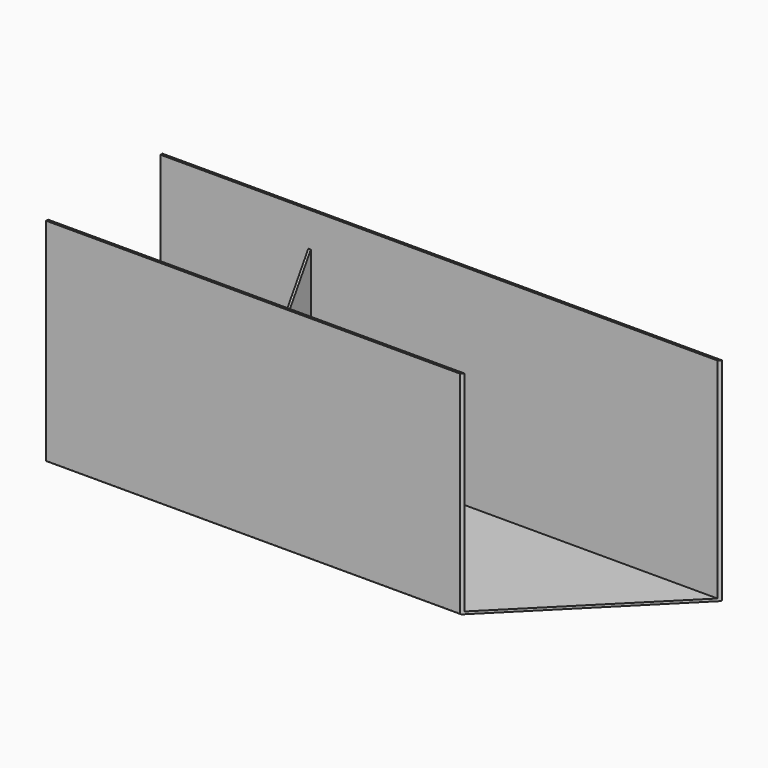
from build123d import *

# Parameters (mm, degrees)
F1_DEPTH = 1200
F4_DEPTH = 5
F5_W     = 1200
F5_H     = 230
F6_DEPTH = 4
F7_R     = 2
F9_DEPTH = 430.001


# Not quite as in the source:
# - a feature names something its author has since deleted; it is built from what else it names


with BuildPart() as f1:
    # F0 (on Right) → F1 (new body)
    with BuildSketch(Plane.YZ):
        Polygon((-295, 0), (0, 0), (0, 430), (-5, 430), (-5, 5), (-290, 5), (-290, 430), (-295, 430), align=None)
    extrude(amount=F1_DEPTH)



with BuildPart() as f4:
    # F3 (on offset) → F4 (new body)
    with BuildSketch(Plane.YZ.offset(300)):
        Polygon((-230, 0), (-5, 0), (-5, 360), align=None)
    extrude(amount=F4_DEPTH)


with BuildPart() as f1_1:
    add(f1.part)

    add(f4.part)  # F6 merges F4
    # F5 (on Top) → F6 (join)
    with BuildSketch(Plane.XY):
        with Locations((600, -115)):
            Rectangle(F5_W, F5_H)
    extrude(amount=F6_DEPTH)

    # F7
    f7_edges = [f1_1.edges().sort_by_distance(p)[0] for p in [
        (600, 0, 0),
        (600, -295, 0),
    ]]
    fillet(f7_edges, radius=F7_R)

    # F8 (on face) → F9 (cut, through all)
    with BuildSketch(Plane.XY.offset(430)):
        Polygon((1135, 0), (840, -295), (1200, -295), (1200, 0), align=None)
    extrude(amount=-F9_DEPTH, mode=Mode.SUBTRACT)


solid = f1_1.part
